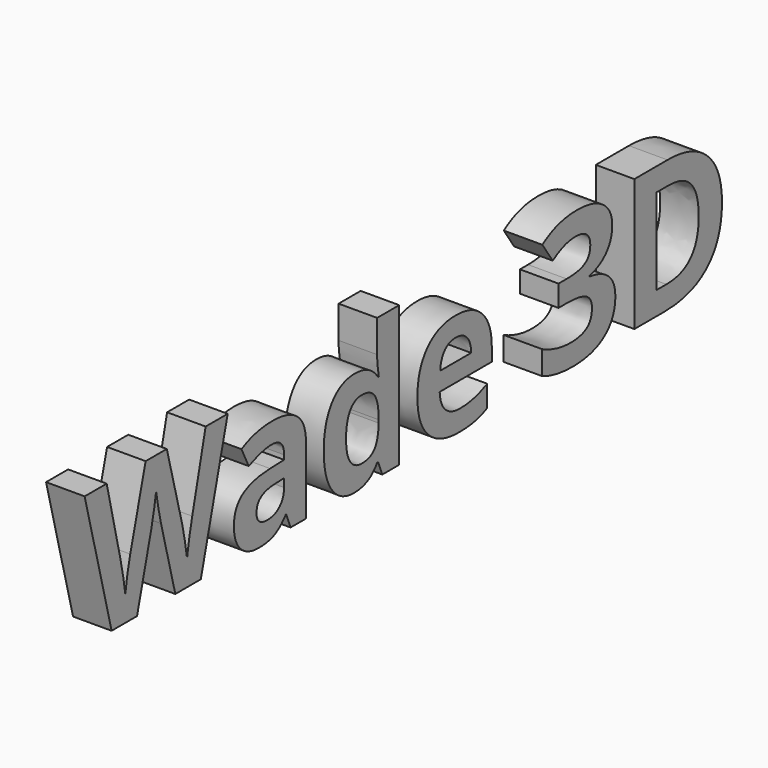
from build123d import *

# Parameters (mm, degrees)
F0_TEXT_SIZE = 121.8122423678
F1_DEPTH     = 25.4


# Not quite as in the source:
# - Text() gives the source's letters only with a copy of the font that has no kerning and outlines rounded to 1/6400 em; it was checked with that copy


with BuildPart() as f1:
    # F0 (on Right) → F1 (new body)
    with BuildSketch(Plane.YZ):
        with Locations((-183.4794133902, -4.0657813661)):
            Text('Wade 3D', F0_TEXT_SIZE, font='Open Sans', font_style=FontStyle.BOLD, text_align=(TextAlign.LEFT, TextAlign.BOTTOM))
    extrude(amount=F1_DEPTH)


solid = f1.part
